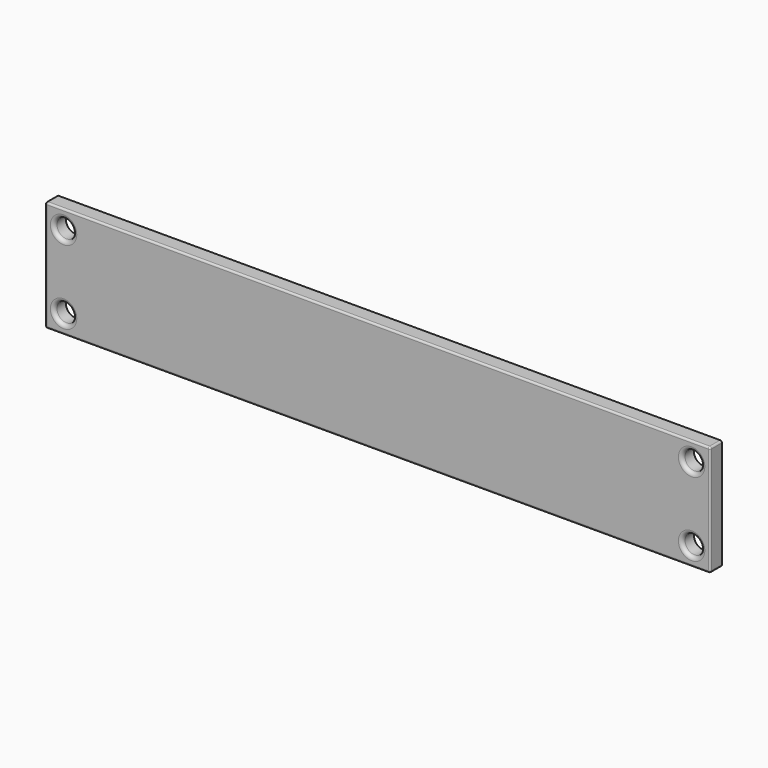
from build123d import *

# Parameters (mm, degrees)
F0_W     = 180
F0_H     = 30
F0_R     = 2.5751263091
F1_DEPTH = 4
F2_R     = 1
F3_R     = 0.5


# Not quite as in the source:
# - a feature names something its author has since deleted; it is built from what else it names


with BuildPart() as f1:
    # F0 (on Front) → F1 (new body)
    with BuildSketch(Plane.XZ):
        Rectangle(F0_W, F0_H)
        with Locations((-85, -10)):
            Circle(F0_R, mode=Mode.SUBTRACT)
        with Locations((85, -10)):
            Circle(F0_R, mode=Mode.SUBTRACT)
        with Locations((-85, 10)):
            Circle(F0_R, mode=Mode.SUBTRACT)
        with Locations((85, 10)):
            Circle(F0_R, mode=Mode.SUBTRACT)
    extrude(amount=F1_DEPTH)

    # F2
    f2_edges = [f1.edges().sort_by_distance(p)[0] for p in [
        (-87.575126, -4, 10),
        (-87.575126, -4, -10),
        (82.424874, -4, 10),
        (82.424874, -4, -10),
    ]]
    fillet(f2_edges, radius=F2_R)

    # F3
    f3_edges = [f1.edges().sort_by_distance(p)[0] for p in [
        (0, -4, 15),
        (-90, -4, 0),
        (0, -4, -15),
        (90, -4, 0),
        (-90, -2, 15),
        (-90, -2, -15),
        (90, -2, 15),
        (90, -2, -15),
    ]]
    fillet(f3_edges, radius=F3_R)


solid = f1.part
